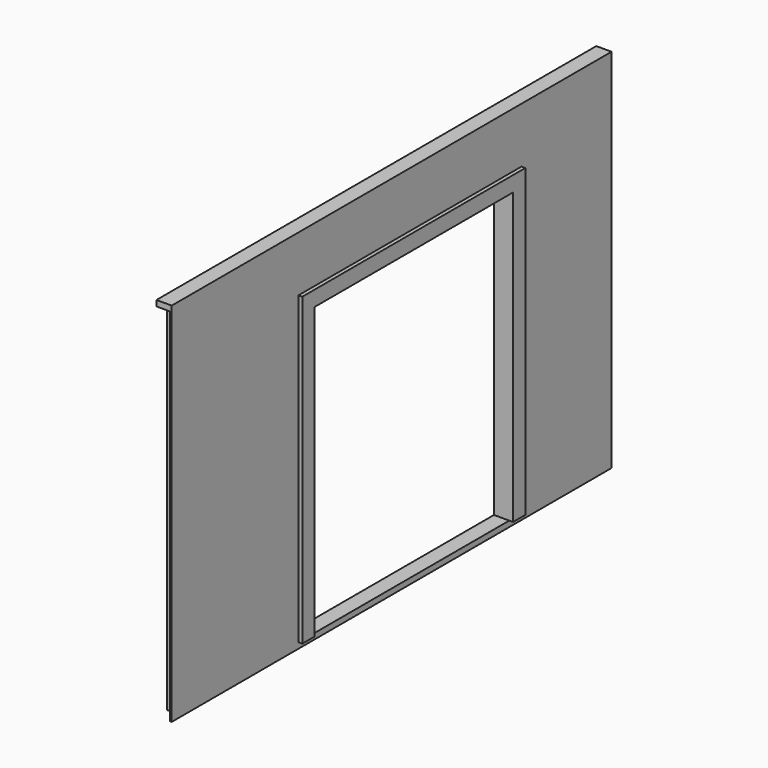
from build123d import *

# Parameters (mm, degrees)
F0_W     = 38.1
F0_H     = 2324.1
F0_H_2   = 1930.4
F1_DEPTH = 88.9
F2_W     = 3657.6
F2_H     = 2438.4
F2_W_2   = 1651
F2_H_2   = 1930.4
F3_DEPTH = 12.7
F5_DEPTH = 25.4


# Not quite as in the source:
# - a feature names something its author has since deleted; it is built from what else it names


with BuildPart() as f1:
    # F0 (on Right) → F1 (new body)
    with BuildSketch(Plane.YZ):
        with Locations((19.05, 1200.15)):
            Rectangle(F0_W, F0_H)
        with Locations((361.95, 1200.15)):
            Rectangle(F0_W, F0_H)
        Polygon((990.6, 2362.2), (990.6, 38.1), (1028.7, 38.1), (1028.7, 1968.5), (1028.7, 2108.2), (1028.7, 2362.2), align=None)
        with Locations((1047.75, 1003.3)):
            Rectangle(F0_W, F0_H_2)
        Polygon((2717.8, 1968.5), (2755.9, 1968.5), (2755.9, 2108.2), (1028.7, 2108.2), (1028.7, 1968.5), (1066.8, 1968.5), align=None)
        with Locations((2736.85, 1003.3)):
            Rectangle(F0_W, F0_H_2)
        Polygon((2755.9, 38.1), (2794, 38.1), (2794, 2362.2), (2755.9, 2362.2), (2755.9, 2108.2), (2755.9, 1968.5), align=None)
        with Locations((3460.75, 1200.15)):
            Rectangle(F0_W, F0_H)
        Polygon((0, 2400.3), (0, 2362.2), (38.1, 2362.2), (342.9, 2362.2), (381, 2362.2), (685.8, 2362.2), (723.9, 2362.2), (990.6, 2362.2), (1028.7, 2362.2), (2755.9, 2362.2), (2794, 2362.2), (3098.8, 2362.2), (3136.9, 2362.2), (3441.7, 2362.2), (3479.8, 2362.2), (3479.8, 2400.3), align=None)
        Polygon((-88.9, 2400.3), (0, 2400.3), (3479.8, 2400.3), (3568.7, 2400.3), (3568.7, 2438.4), (-88.9, 2438.4), align=None)
        Polygon((0, 38.1), (0, 0), (3479.8, 0), (3479.8, 38.1), (3441.7, 38.1), (3136.9, 38.1), (3098.8, 38.1), (2794, 38.1), (2755.9, 38.1), (2717.8, 38.1), (1066.8, 38.1), (1028.7, 38.1), (990.6, 38.1), (723.9, 38.1), (685.8, 38.1), (381, 38.1), (342.9, 38.1), (38.1, 38.1), align=None)
        with Locations((704.85, 1200.15)):
            Rectangle(F0_W, F0_H)
        with Locations((3117.85, 1200.15)):
            Rectangle(F0_W, F0_H)
    extrude(amount=F1_DEPTH)

    # F2 (on face) → F3 (join)
    with BuildSketch(Plane.YZ.offset(88.9)):
        with Locations((1739.9, 1219.2)):
            Rectangle(F2_W, F2_H)
        with Locations((1892.3, 1003.3)):
            Rectangle(F2_W_2, F2_H_2, mode=Mode.SUBTRACT)
    extrude(amount=F3_DEPTH)

    # F4 (on face) → F5 (join)
    with BuildSketch(Plane.YZ.offset(101.6)):
        Polygon((1066.8, 38.1), (1066.8, 1968.5), (2717.8, 1968.5), (2717.8, 38.1), (2819.4, 38.1), (2819.4, 2070.1), (965.2, 2070.1), (965.2, 38.1), align=None)
    extrude(amount=F5_DEPTH)


solid = f1.part
